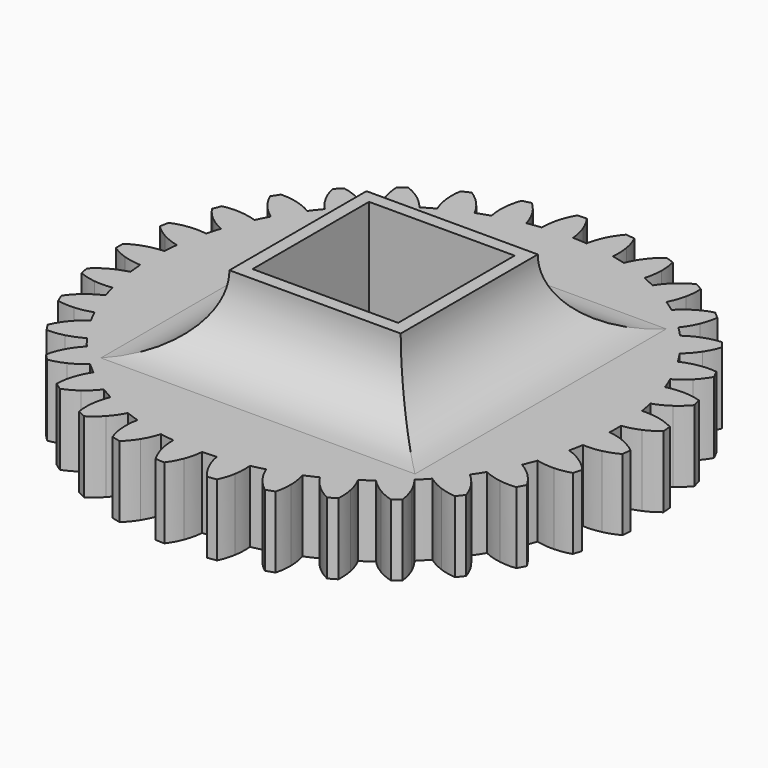
from build123d import *

# Parameters (mm, degrees)
F1_DEPTH = 5
F2_COUNT = 33
F3_W     = 10.2
F3_H     = 10.2
F4_DEPTH = 6
F3_W_2   = 12
F3_H_2   = 12
F5_DEPTH = 5
F6_R     = 4.99999


# Not quite as in the source:
# - a fillet or chamfer is up to 0.001 mm smaller than in the source, because OpenCascade refuses the exact size


with BuildPart() as f1:
    # F0 (on Top) → F1 (new body)
    with BuildSketch(Plane.XY):
        with BuildLine():
            ThreePointArc((-1.8233572605, 16.1354794051), (-10.8182792774, -12.1096309113), (16.238175, 0))
            ThreePointArc((16.238175, 0), (11.5811549349, 11.3822307877), (0.2813106722, 16.2357380995))
            ThreePointArc((0.2813106722, 16.2357380995), (-0.7726511966, 16.2197822877), (-1.8233572605, 16.1354794051))
        make_face()
        with BuildLine():
            ThreePointArc((-1.8233572605, 16.1354794051), (-0.7726511966, 16.2197822877), (0.2813106722, 16.2357380995))
            ThreePointArc((0.2813106722, 16.2357380995), (0.18304777, 16.8588401245), (0, 17.4625))
            ThreePointArc((0, 17.4625), (-0.2474169209, 17.9997398777), (-0.5655469096, 18.4983731389))
            ThreePointArc((-0.5655469096, 18.4983731389), (-0.880518131, 18.4841652322), (-1.1954136706, 18.4683685865))
            ThreePointArc((-1.1954136706, 18.4683685865), (-1.4647045359, 17.941752741), (-1.6599327052, 17.3834268677))
            ThreePointArc((-1.6599327052, 17.3834268677), (-1.7847695128, 16.7651004952), (-1.8233572605, 16.1354794051))
        make_face()
    extrude(amount=F1_DEPTH)


with BuildPart() as f2_1:
    # F2: instance of F1
    add(f1.part.rotate(Axis((0, 0, 0), (0, 0, -1)), 1 * 360 / F2_COUNT))


with BuildPart() as f2_2:
    # F2: instance of F1
    add(f1.part.rotate(Axis((0, 0, 0), (0, 0, -1)), 2 * 360 / F2_COUNT))


with BuildPart() as f2_3:
    # F2: instance of F1
    add(f1.part.rotate(Axis((0, 0, 0), (0, 0, -1)), 3 * 360 / F2_COUNT))


with BuildPart() as f2_4:
    # F2: instance of F1
    add(f1.part.rotate(Axis((0, 0, 0), (0, 0, -1)), 4 * 360 / F2_COUNT))


with BuildPart() as f2_5:
    # F2: instance of F1
    add(f1.part.rotate(Axis((0, 0, 0), (0, 0, -1)), 5 * 360 / F2_COUNT))


with BuildPart() as f2_6:
    # F2: instance of F1
    add(f1.part.rotate(Axis((0, 0, 0), (0, 0, -1)), 6 * 360 / F2_COUNT))


with BuildPart() as f2_7:
    # F2: instance of F1
    add(f1.part.rotate(Axis((0, 0, 0), (0, 0, -1)), 7 * 360 / F2_COUNT))


with BuildPart() as f2_8:
    # F2: instance of F1
    add(f1.part.rotate(Axis((0, 0, 0), (0, 0, -1)), 8 * 360 / F2_COUNT))


with BuildPart() as f2_9:
    # F2: instance of F1
    add(f1.part.rotate(Axis((0, 0, 0), (0, 0, -1)), 9 * 360 / F2_COUNT))


with BuildPart() as f2_10:
    # F2: instance of F1
    add(f1.part.rotate(Axis((0, 0, 0), (0, 0, -1)), 10 * 360 / F2_COUNT))


with BuildPart() as f2_11:
    # F2: instance of F1
    add(f1.part.rotate(Axis((0, 0, 0), (0, 0, -1)), 11 * 360 / F2_COUNT))


with BuildPart() as f2_12:
    # F2: instance of F1
    add(f1.part.rotate(Axis((0, 0, 0), (0, 0, -1)), 12 * 360 / F2_COUNT))


with BuildPart() as f2_13:
    # F2: instance of F1
    add(f1.part.rotate(Axis((0, 0, 0), (0, 0, -1)), 13 * 360 / F2_COUNT))


with BuildPart() as f2_14:
    # F2: instance of F1
    add(f1.part.rotate(Axis((0, 0, 0), (0, 0, -1)), 14 * 360 / F2_COUNT))


with BuildPart() as f2_15:
    # F2: instance of F1
    add(f1.part.rotate(Axis((0, 0, 0), (0, 0, -1)), 15 * 360 / F2_COUNT))


with BuildPart() as f2_16:
    # F2: instance of F1
    add(f1.part.rotate(Axis((0, 0, 0), (0, 0, -1)), 16 * 360 / F2_COUNT))


with BuildPart() as f2_17:
    # F2: instance of F1
    add(f1.part.rotate(Axis((0, 0, 0), (0, 0, -1)), 17 * 360 / F2_COUNT))


with BuildPart() as f2_18:
    # F2: instance of F1
    add(f1.part.rotate(Axis((0, 0, 0), (0, 0, -1)), 18 * 360 / F2_COUNT))


with BuildPart() as f2_19:
    # F2: instance of F1
    add(f1.part.rotate(Axis((0, 0, 0), (0, 0, -1)), 19 * 360 / F2_COUNT))


with BuildPart() as f2_20:
    # F2: instance of F1
    add(f1.part.rotate(Axis((0, 0, 0), (0, 0, -1)), 20 * 360 / F2_COUNT))


with BuildPart() as f2_21:
    # F2: instance of F1
    add(f1.part.rotate(Axis((0, 0, 0), (0, 0, -1)), 21 * 360 / F2_COUNT))


with BuildPart() as f2_22:
    # F2: instance of F1
    add(f1.part.rotate(Axis((0, 0, 0), (0, 0, -1)), 22 * 360 / F2_COUNT))


with BuildPart() as f2_23:
    # F2: instance of F1
    add(f1.part.rotate(Axis((0, 0, 0), (0, 0, -1)), 23 * 360 / F2_COUNT))


with BuildPart() as f2_24:
    # F2: instance of F1
    add(f1.part.rotate(Axis((0, 0, 0), (0, 0, -1)), 24 * 360 / F2_COUNT))


with BuildPart() as f2_25:
    # F2: instance of F1
    add(f1.part.rotate(Axis((0, 0, 0), (0, 0, -1)), 25 * 360 / F2_COUNT))


with BuildPart() as f2_26:
    # F2: instance of F1
    add(f1.part.rotate(Axis((0, 0, 0), (0, 0, -1)), 26 * 360 / F2_COUNT))


with BuildPart() as f2_27:
    # F2: instance of F1
    add(f1.part.rotate(Axis((0, 0, 0), (0, 0, -1)), 27 * 360 / F2_COUNT))


with BuildPart() as f2_28:
    # F2: instance of F1
    add(f1.part.rotate(Axis((0, 0, 0), (0, 0, -1)), 28 * 360 / F2_COUNT))


with BuildPart() as f2_29:
    # F2: instance of F1
    add(f1.part.rotate(Axis((0, 0, 0), (0, 0, -1)), 29 * 360 / F2_COUNT))


with BuildPart() as f2_30:
    # F2: instance of F1
    add(f1.part.rotate(Axis((0, 0, 0), (0, 0, -1)), 30 * 360 / F2_COUNT))


with BuildPart() as f2_31:
    # F2: instance of F1
    add(f1.part.rotate(Axis((0, 0, 0), (0, 0, -1)), 31 * 360 / F2_COUNT))


with BuildPart() as f2_32:
    # F2: instance of F1
    add(f1.part.rotate(Axis((0, 0, 0), (0, 0, -1)), 32 * 360 / F2_COUNT))


with BuildPart() as f4_tool:
    # F3 (on face) → F4 (new body)
    with BuildSketch(Plane.XY.offset(5)):
        Rectangle(F3_W, F3_H)
    extrude(amount=-F4_DEPTH)


with BuildPart() as f1_1:
    add(f1.part)

    # F4: cut by f4_tool
    add(f4_tool.part, mode=Mode.SUBTRACT)



with BuildPart() as f2_1_1:
    add(f2_1.part)

    # F4: cut by f4_tool
    add(f4_tool.part, mode=Mode.SUBTRACT)


with BuildPart() as f2_2_1:
    add(f2_2.part)

    # F4: cut by f4_tool
    add(f4_tool.part, mode=Mode.SUBTRACT)


with BuildPart() as f2_3_1:
    add(f2_3.part)

    # F4: cut by f4_tool
    add(f4_tool.part, mode=Mode.SUBTRACT)


with BuildPart() as f2_4_1:
    add(f2_4.part)

    # F4: cut by f4_tool
    add(f4_tool.part, mode=Mode.SUBTRACT)


with BuildPart() as f2_5_1:
    add(f2_5.part)

    # F4: cut by f4_tool
    add(f4_tool.part, mode=Mode.SUBTRACT)


with BuildPart() as f2_6_1:
    add(f2_6.part)

    # F4: cut by f4_tool
    add(f4_tool.part, mode=Mode.SUBTRACT)


with BuildPart() as f2_7_1:
    add(f2_7.part)

    # F4: cut by f4_tool
    add(f4_tool.part, mode=Mode.SUBTRACT)


with BuildPart() as f2_8_1:
    add(f2_8.part)

    # F4: cut by f4_tool
    add(f4_tool.part, mode=Mode.SUBTRACT)


with BuildPart() as f2_9_1:
    add(f2_9.part)

    # F4: cut by f4_tool
    add(f4_tool.part, mode=Mode.SUBTRACT)


with BuildPart() as f2_10_1:
    add(f2_10.part)

    # F4: cut by f4_tool
    add(f4_tool.part, mode=Mode.SUBTRACT)


with BuildPart() as f2_11_1:
    add(f2_11.part)

    # F4: cut by f4_tool
    add(f4_tool.part, mode=Mode.SUBTRACT)


with BuildPart() as f2_12_1:
    add(f2_12.part)

    # F4: cut by f4_tool
    add(f4_tool.part, mode=Mode.SUBTRACT)


with BuildPart() as f2_13_1:
    add(f2_13.part)

    # F4: cut by f4_tool
    add(f4_tool.part, mode=Mode.SUBTRACT)


with BuildPart() as f2_14_1:
    add(f2_14.part)

    # F4: cut by f4_tool
    add(f4_tool.part, mode=Mode.SUBTRACT)


with BuildPart() as f2_15_1:
    add(f2_15.part)

    # F4: cut by f4_tool
    add(f4_tool.part, mode=Mode.SUBTRACT)


with BuildPart() as f2_16_1:
    add(f2_16.part)

    # F4: cut by f4_tool
    add(f4_tool.part, mode=Mode.SUBTRACT)


with BuildPart() as f2_17_1:
    add(f2_17.part)

    # F4: cut by f4_tool
    add(f4_tool.part, mode=Mode.SUBTRACT)


with BuildPart() as f2_18_1:
    add(f2_18.part)

    # F4: cut by f4_tool
    add(f4_tool.part, mode=Mode.SUBTRACT)


with BuildPart() as f2_19_1:
    add(f2_19.part)

    # F4: cut by f4_tool
    add(f4_tool.part, mode=Mode.SUBTRACT)


with BuildPart() as f2_20_1:
    add(f2_20.part)

    # F4: cut by f4_tool
    add(f4_tool.part, mode=Mode.SUBTRACT)


with BuildPart() as f2_21_1:
    add(f2_21.part)

    # F4: cut by f4_tool
    add(f4_tool.part, mode=Mode.SUBTRACT)


with BuildPart() as f2_22_1:
    add(f2_22.part)

    # F4: cut by f4_tool
    add(f4_tool.part, mode=Mode.SUBTRACT)


with BuildPart() as f2_23_1:
    add(f2_23.part)

    # F4: cut by f4_tool
    add(f4_tool.part, mode=Mode.SUBTRACT)


with BuildPart() as f2_24_1:
    add(f2_24.part)

    # F4: cut by f4_tool
    add(f4_tool.part, mode=Mode.SUBTRACT)


with BuildPart() as f2_25_1:
    add(f2_25.part)

    # F4: cut by f4_tool
    add(f4_tool.part, mode=Mode.SUBTRACT)


with BuildPart() as f2_26_1:
    add(f2_26.part)

    # F4: cut by f4_tool
    add(f4_tool.part, mode=Mode.SUBTRACT)


with BuildPart() as f2_27_1:
    add(f2_27.part)

    # F4: cut by f4_tool
    add(f4_tool.part, mode=Mode.SUBTRACT)


with BuildPart() as f2_28_1:
    add(f2_28.part)

    # F4: cut by f4_tool
    add(f4_tool.part, mode=Mode.SUBTRACT)


with BuildPart() as f2_29_1:
    add(f2_29.part)

    # F4: cut by f4_tool
    add(f4_tool.part, mode=Mode.SUBTRACT)


with BuildPart() as f2_30_1:
    add(f2_30.part)

    # F4: cut by f4_tool
    add(f4_tool.part, mode=Mode.SUBTRACT)


with BuildPart() as f2_31_1:
    add(f2_31.part)

    # F4: cut by f4_tool
    add(f4_tool.part, mode=Mode.SUBTRACT)


with BuildPart() as f2_32_1:
    add(f2_32.part)

    # F4: cut by f4_tool
    add(f4_tool.part, mode=Mode.SUBTRACT)


with BuildPart() as f1_2:
    add(f1_1.part)

    add(f2_1_1.part)  # F5 merges F2_1

    add(f2_2_1.part)  # F5 merges F2_2

    add(f2_3_1.part)  # F5 merges F2_3

    add(f2_4_1.part)  # F5 merges F2_4

    add(f2_5_1.part)  # F5 merges F2_5

    add(f2_6_1.part)  # F5 merges F2_6

    add(f2_7_1.part)  # F5 merges F2_7

    add(f2_8_1.part)  # F5 merges F2_8

    add(f2_9_1.part)  # F5 merges F2_9

    add(f2_10_1.part)  # F5 merges F2_10

    add(f2_11_1.part)  # F5 merges F2_11

    add(f2_12_1.part)  # F5 merges F2_12

    add(f2_13_1.part)  # F5 merges F2_13

    add(f2_14_1.part)  # F5 merges F2_14

    add(f2_15_1.part)  # F5 merges F2_15

    add(f2_16_1.part)  # F5 merges F2_16

    add(f2_17_1.part)  # F5 merges F2_17

    add(f2_18_1.part)  # F5 merges F2_18

    add(f2_19_1.part)  # F5 merges F2_19

    add(f2_20_1.part)  # F5 merges F2_20

    add(f2_21_1.part)  # F5 merges F2_21

    add(f2_22_1.part)  # F5 merges F2_22

    add(f2_23_1.part)  # F5 merges F2_23

    add(f2_24_1.part)  # F5 merges F2_24

    add(f2_25_1.part)  # F5 merges F2_25

    add(f2_26_1.part)  # F5 merges F2_26

    add(f2_27_1.part)  # F5 merges F2_27

    add(f2_28_1.part)  # F5 merges F2_28

    add(f2_29_1.part)  # F5 merges F2_29

    add(f2_30_1.part)  # F5 merges F2_30

    add(f2_31_1.part)  # F5 merges F2_31

    add(f2_32_1.part)  # F5 merges F2_32
    # F3 (on face) → F5 (join)
    with BuildSketch(Plane.XY.offset(5)):
        Rectangle(F3_W_2, F3_H_2)
        Rectangle(F3_W, F3_H, mode=Mode.SUBTRACT)
    extrude(amount=F5_DEPTH)

    # F6 (radius 5 in the source; OpenCascade refuses exactly that, so slightly less here)
    f6_edges = [f1_2.edges().sort_by_distance(p)[0] for p in [
        (0, -6, 5),
        (-6, 0, 5),
        (0, 6, 5),
        (6, 0, 5),
    ]]
    fillet(f6_edges, radius=F6_R)


solid = f1_2.part
